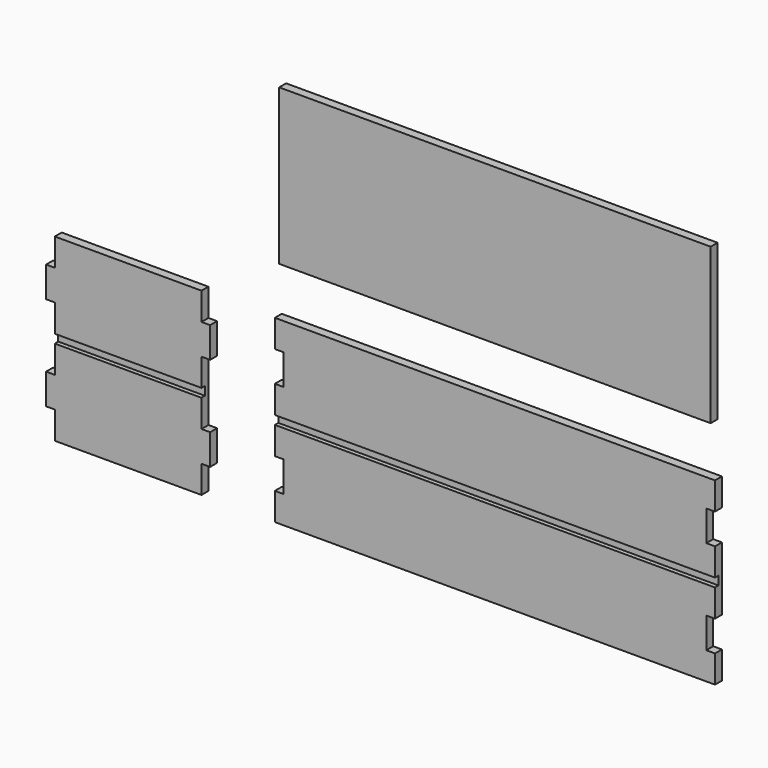
from build123d import *

# Parameters (mm, degrees)
F1_W     = 18.034
F1_H     = 63.5
F2_DEPTH = 18.034
F1_W_2   = 896.366
F1_H_2   = 322.834
F1_W_3   = 304.8
F1_H_3   = 18.034
F3_DEPTH = 9.017
F1_W_4   = 914.4


# Not quite as in the source:
# - a variable given as a bare number and used for a length is read in inches; the dataset says mm whatever the document's units were
# - a feature names something its author has since deleted; it is built from what else it names


with BuildPart() as f2:
    # F1 (on Front) → F2 (new body)
    with BuildSketch(Plane.XZ):
        Polygon((-609.6, 129.667), (-609.6, 186.817), (-914.4, 186.817), (-914.4, 129.667), (-914.4, 66.167), (-914.4, 9.017), (-609.6, 9.017), (-609.6, 66.167), align=None)
        with Locations((-923.417, 97.917)):
            Rectangle(F1_W, F1_H)
        with Locations((-600.583, 97.917)):
            Rectangle(F1_W, F1_H)
    extrude(amount=F2_DEPTH)



with BuildPart() as f2b:
    # F1 (on Front) → F2, piece 2 (new body)
    with BuildSketch(Plane.XZ):
        with Locations((-923.417, -97.917)):
            Rectangle(F1_W, F1_H)
        with Locations((-600.583, -97.917)):
            Rectangle(F1_W, F1_H)
        Polygon((-609.6, -66.167), (-609.6, -9.017), (-914.4, -9.017), (-914.4, -66.167), (-914.4, -129.667), (-914.4, -186.817), (-609.6, -186.817), (-609.6, -129.667), align=None)
    extrude(amount=F2_DEPTH)


with BuildPart() as f2c:
    # F1 (on Front) → F2, piece 3 (new body)
    with BuildSketch(Plane.XZ):
        Polygon((457.2, -9.017), (-457.2, -9.017), (-457.2, -66.167), (-439.166, -66.167), (-439.166, -129.667), (-457.2, -129.667), (-457.2, -186.817), (457.2, -186.817), (457.2, -129.667), (439.166, -129.667), (439.166, -66.167), (457.2, -66.167), align=None)
    extrude(amount=F2_DEPTH)



with BuildPart() as f2d:
    # F1 (on Front) → F2, piece 4 (new body)
    with BuildSketch(Plane.XZ):
        Polygon((457.2, 186.817), (-457.2, 186.817), (-457.2, 129.667), (-439.166, 129.667), (-439.166, 66.167), (-457.2, 66.167), (-457.2, 9.017), (457.2, 9.017), (457.2, 66.167), (439.166, 66.167), (439.166, 129.667), (457.2, 129.667), align=None)
    extrude(amount=F2_DEPTH)


with BuildPart() as f2e:
    # F1 (on Front) → F2, piece 5 (new body)
    with BuildSketch(Plane.XZ):
        with Locations((0, 449.834)):
            Rectangle(F1_W_2, F1_H_2)
    extrude(amount=F2_DEPTH)


with BuildPart() as f2_1:
    add(f2.part)

    add(f2b.part)  # F3 merges F2b
    # F1 (on Front) → F3 (join)
    with BuildSketch(Plane.XZ):
        with Locations((-762, 0)):
            Rectangle(F1_W_3, F1_H_3)
    extrude(amount=F3_DEPTH)


with BuildPart() as f2c_1:
    add(f2c.part)

    add(f2d.part)  # F3#2 merges F2d
    # F1 (on Front) → F3, piece 2 (join)
    with BuildSketch(Plane.XZ):
        Rectangle(F1_W_4, F1_H_3)
    extrude(amount=F3_DEPTH)


solid = Compound([f2e.part, f2_1.part, f2c_1.part])
